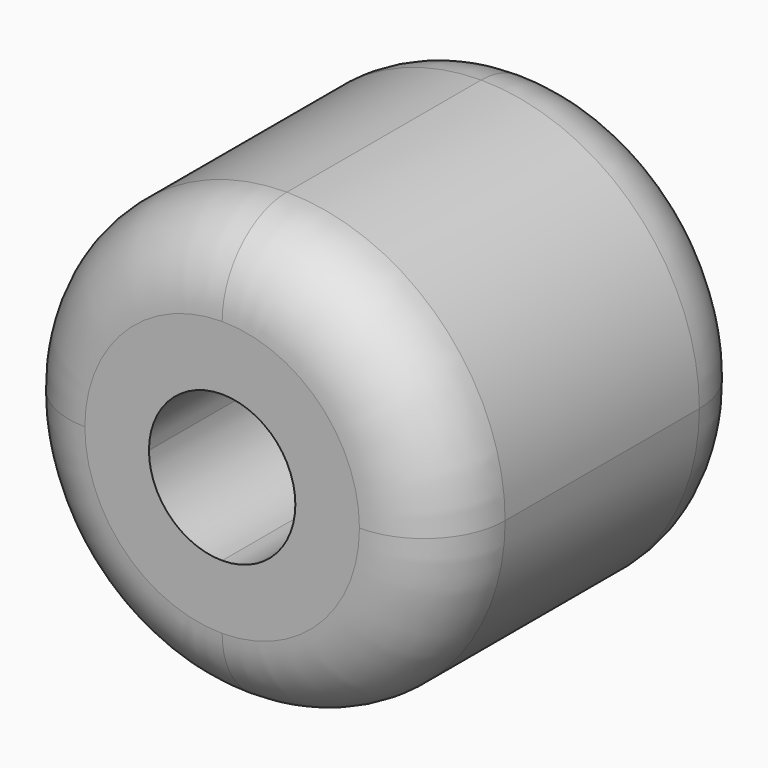
from build123d import *

# Parameters (mm, degrees)
F1_DEPTH = 12.7
F2_R     = 5.08


with BuildPart() as f1:
    # F0 (on Front) → F1 (new body, symmetric)
    with BuildSketch(Plane.XZ):
        with BuildLine():
            Line((4.595115, 0), (13.699897, 0))
            ThreePointArc((13.699897, 0), (9.68729, 9.68729), (0, 13.699897))
            Line((0, 13.699897), (0, 4.595115))
            ThreePointArc((0, 4.595115), (3.249237, 3.249237), (4.595115, 0))
        make_face()
        with BuildLine():
            Line((0, 4.595115), (0, 13.699897))
            ThreePointArc((0, 13.699897), (-9.68729, 9.68729), (-13.699897, 0))
            Line((-13.699897, 0), (-4.595115, 0))
            ThreePointArc((-4.595115, 0), (-3.249237, 3.249237), (0, 4.595115))
        make_face()
        with BuildLine():
            ThreePointArc((0, -13.699897), (9.68729, -9.68729), (13.699897, 0))
            Line((13.699897, 0), (4.595115, 0))
            ThreePointArc((4.595115, 0), (3.249237, -3.249237), (0, -4.595115))
            Line((0, -4.595115), (0, -13.699897))
        make_face()
        with BuildLine():
            ThreePointArc((-13.699897, 0), (-9.68729, -9.68729), (0, -13.699897))
            Line((0, -13.699897), (0, -4.595115))
            ThreePointArc((0, -4.595115), (-3.249237, -3.249237), (-4.595115, 0))
            Line((-4.595115, 0), (-13.699897, 0))
        make_face()
    extrude(amount=F1_DEPTH, both=True)

    # F2
    f2_edges = [f1.edges().sort_by_distance(p)[0] for p in [
        (13.699897, -12.7, 0),
        (13.699897, 12.7, 0),
    ]]
    fillet(f2_edges, radius=F2_R)


solid = f1.part
